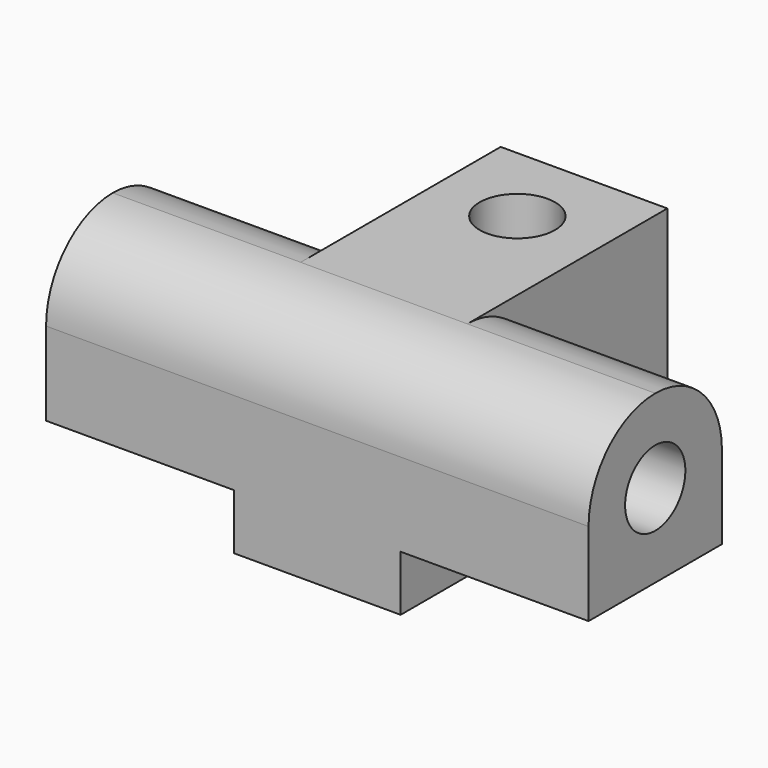
from build123d import *

# Parameters (mm, degrees)
F0_W     = 31
F0_H     = 19.05
F0_R     = 2.15265
F1_DEPTH = 9.525
F2_R     = 2.15265
F3_DEPTH = 31
F4_W     = 9.525
F4_H     = 9.525
F5_DEPTH = 3.175
F6_W     = 10.7375
F6_H     = 9.525
F7_DEPTH = 9.525
F8_R     = 4.76249


# Not quite as in the source:
# - a fillet or chamfer is up to 0.001 mm smaller than in the source, because OpenCascade refuses the exact size


with BuildPart() as f1:
    # F0 (on Top) → F1 (new body)
    with BuildSketch(Plane.XY):
        with Locations((15.5, -9.525)):
            Rectangle(F0_W, F0_H)
        with Locations((15.5, -4.7625)):
            Circle(F0_R, mode=Mode.SUBTRACT)
    extrude(amount=F1_DEPTH)

    # F2 (on face) → F3 (cut, through all)
    with BuildSketch(Plane.YZ.offset(31)):
        with Locations((-14.2875, 4.7625)):
            Circle(F2_R)
    extrude(amount=-F3_DEPTH, mode=Mode.SUBTRACT)

    # F4 (on face) → F5 (join)
    with BuildSketch(Plane(origin=(0, 0, 0), x_dir=(1, 0, 0), z_dir=(0, 0, -1))):
        with Locations((15.5, 14.2875)):
            Rectangle(F4_W, F4_H)
    extrude(amount=F5_DEPTH)

    # F6 (on face) → F7 (cut, through all)
    with BuildSketch(Plane(origin=(0, 0, 0), x_dir=(1, 0, 0), z_dir=(0, 0, -1))):
        with Locations((25.63125, 4.7625)):
            Rectangle(F6_W, F6_H)
        with Locations((5.36875, 4.7625)):
            Rectangle(F6_W, F6_H)
    extrude(amount=-F7_DEPTH, mode=Mode.SUBTRACT)

    # F8 (radius 4.7625 in the source; OpenCascade refuses exactly that, so slightly less here)
    f8_edges = [f1.edges().sort_by_distance(p)[0] for p in [
        (15.5, -19.05, 9.525),
        (25.63125, -9.525, 9.525),
        (5.36875, -9.525, 9.525),
    ]]
    fillet(f8_edges, radius=F8_R)


solid = f1.part
